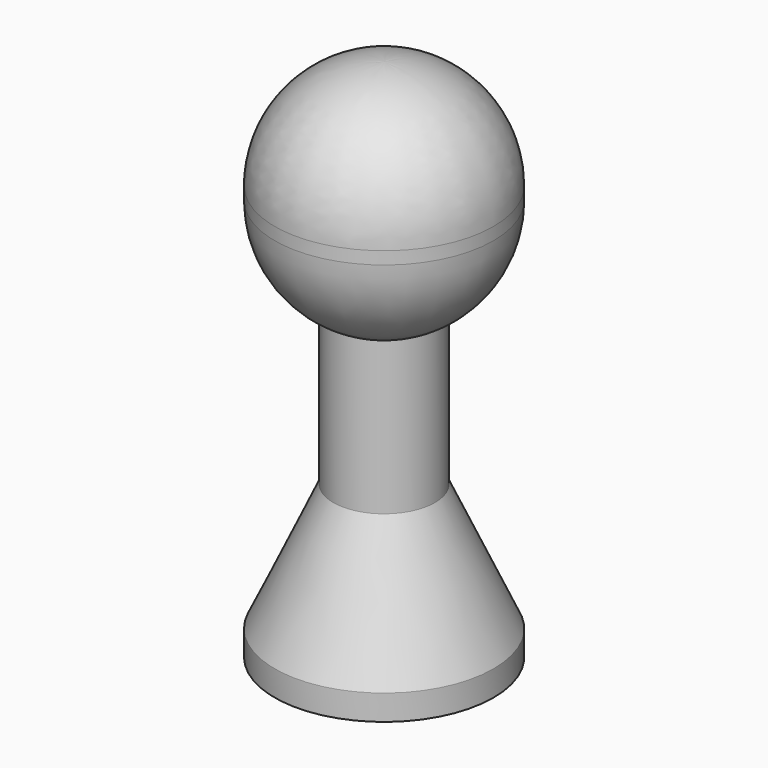
from build123d import *

# Parameters (mm, degrees)
F0_R     = 21.5
F1_DEPTH = 30
F2_SIZE2 = 25
F2_SIZE  = 11.5
F3_DEPTH = 30
F4_R     = 21.5
F5_DEPTH = 43


# Not quite as in the source:
# - a fillet or chamfer that OpenCascade refuses, or shapes differently, is made with other operations: its cross-section is extruded or revolved along the edge and cut away or added


with BuildPart() as f1:
    # F0 (on Top) → F1 (new body)
    with BuildSketch(Plane.XY):
        Circle(F0_R)
    extrude(amount=F1_DEPTH)

    # F2
    f2_edges = [f1.edges().sort_by_distance(p)[0] for p in [
        (-21.5, 0, 30),
    ]]
    f2_side = f1.faces().sort_by_distance((0, 0, 30))[0]
    chamfer(f2_edges, length=F2_SIZE, length2=F2_SIZE2, reference=f2_side)

    # F3 (add): a face of the model
    f3_faces = [f1.faces().sort_by_distance(p)[0] for p in [
        (0, 0, 30),
    ]]
    extrude(f3_faces, amount=F3_DEPTH)

    # F4 (on face) → F5 (join)
    with BuildSketch(Plane.XY.offset(60)):
        Circle(F4_R)
    extrude(amount=F5_DEPTH)

    # F6: fillet of radius 21.499 on 2 edges, made by hand

    # F6_s1 → F6_t2 (revolve, cut)
    with BuildSketch(Plane.XZ):
        with BuildLine():
            ThreePointArc((21.5, 81.501), (15.2030886887, 96.7030886887), (0.001, 103))
            Line((0.001, 103), (21.5, 103))
            Line((21.5, 103), (21.5, 81.501))
        make_face()
    revolve(axis=Axis((0, 0, 103), (0, 0, 1)), mode=Mode.SUBTRACT)

    # F6_s3 → F6_t4 (revolve, cut)
    with BuildSketch(Plane.XZ):
        with BuildLine():
            ThreePointArc((21.5, 79.0322620831), (18.4017540878, 67.913842681), (10, 60))
            Line((10, 60), (21.5, 60))
            Line((21.5, 60), (21.5, 79.0322620831))
        make_face()
    revolve(axis=Axis((0, 0, 60), (0, 0, 1)), mode=Mode.SUBTRACT)


solid = f1.part
